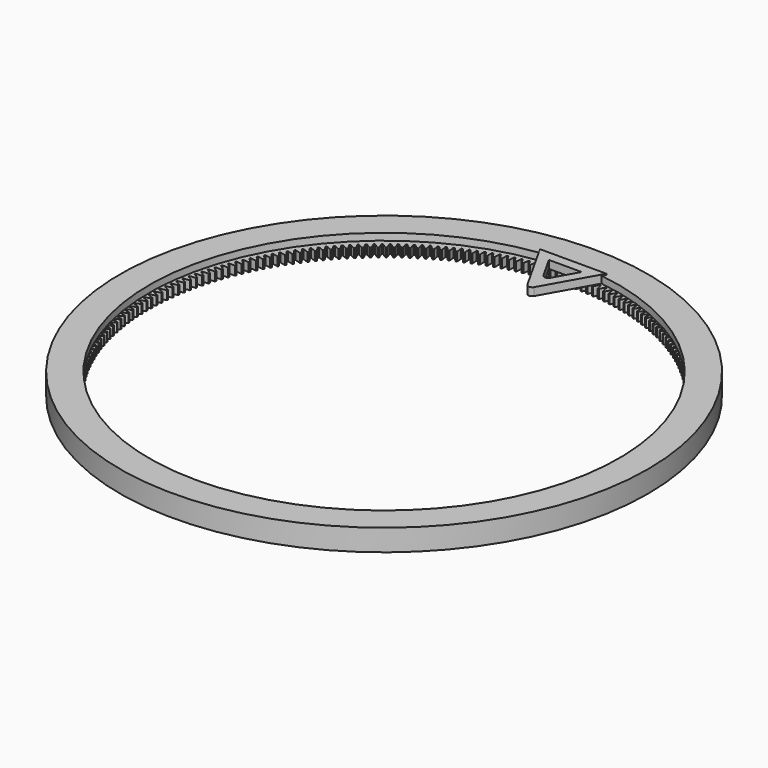
from build123d import *

# Parameters (mm, degrees)
F0_R     = 67
F0_R_2   = 59.6
F1_DEPTH = 3.75
F2_R     = 63.125
F3_DEPTH = 1.5
F4_DEPTH = 2
F6_DEPTH = 6.5
F7_COUNT = 240
F9_DEPTH = 2
F10_R    = 1


with BuildPart() as f1:
    # F0 (on Top) → F1 (new body, symmetric)
    with BuildSketch(Plane.XY):
        Circle(F0_R)
        Circle(F0_R_2, mode=Mode.SUBTRACT)
    extrude(amount=F1_DEPTH, both=True)

    # F2 (on Top) → F3 (cut)
    with BuildSketch(Plane.XY):
        Circle(F2_R)
    extrude(amount=-F3_DEPTH, mode=Mode.SUBTRACT)

    # F4 (cut): a face of the model
    f4_faces = [f1.faces().sort_by_distance(p)[0] for p in [
        (-65.1049538264, 0, 3.75),
    ]]
    extrude(f4_faces, amount=-F4_DEPTH, mode=Mode.SUBTRACT)

    # F5 (on Top) → F6 (cut)
    with BuildSketch(Plane.XY):
        Polygon((61, -0.15), (61, 0.15), (59.4, 0.675), (59.4, -0.675), align=None)
    f6 = extrude(amount=-F6_DEPTH, mode=Mode.SUBTRACT)

    # F7: F6 ×240 about axis
    f7_axis = Axis((0, 0, 0), (0, 0, -1))
    for i in range(1, F7_COUNT):
        add(f6.rotate(f7_axis, i * 360 / F7_COUNT), mode=Mode.SUBTRACT)

    # F8 (on Top) → F9 (join)
    with BuildSketch(Plane.XY):
        Polygon((0, 45), (8.4307833976, 59.988140923), (0, 59.988140923), (-8.4307833976, 59.988140923), align=None)
        Polygon((4.156176089, 57.488140923), (0, 50.0993432295), (-4.156176089, 57.488140923), (0, 57.488140923), align=None, mode=Mode.SUBTRACT)
    extrude(amount=F9_DEPTH)

    # F10
    f10_edges = [f1.edges().sort_by_distance(p)[0] for p in [
        (0, 45, 1),
        (0, 50.099343, 1),
    ]]
    fillet(f10_edges, radius=F10_R)


solid = f1.part
